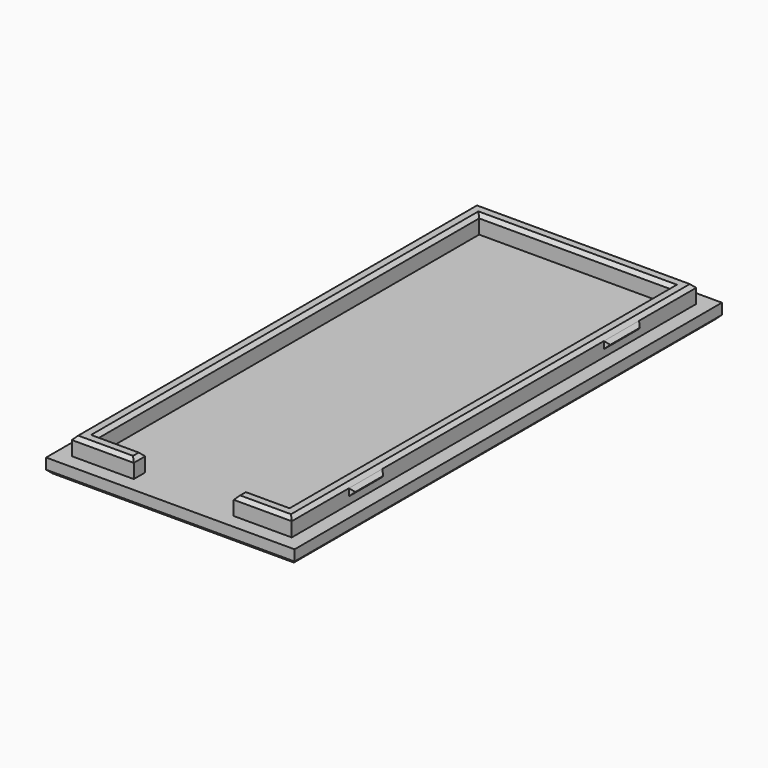
from build123d import *

# Parameters (mm, degrees)
F1_W     = 2
F1_H     = 6.165323171
F1_H_2   = 5.8635988384
F1_H_3   = 38.7710779905
F1_W_2   = 14
F1_H_4   = 2
F1_W_3   = 26.8
F1_H_5   = 8
F1_W_4   = 0.5
F2_DEPTH = 2
F3_START = 1
F3_DEPTH = 3.5
F4_START = 3
F4_DEPTH = 1
F5_SIZE  = 0.49999


# Not quite as in the source:
# - a fillet or chamfer is up to 0.001 mm smaller than in the source, because OpenCascade refuses the exact size


with BuildPart() as f2:
    # F1 (on Top) → F2 (new body)
    with BuildSketch(Plane.XY):
        Polygon((16.0419130247, 37.7546238333), (-14.7580869753, 37.7546238333), (-14.7580869753, 27.7546238333), (-12.7580869753, 27.7546238333), (-12.7580869753, 35.7546238333), (14.0419130247, 35.7546238333), (14.0419130247, 27.7546238333), (16.0419130247, 27.7546238333), align=None)
        Polygon((-12.7580869753, -23.0453761667), (-14.7580869753, -23.0453761667), (-14.7580869753, -26.0453761667), (-14.7580869753, -33.0453761667), (-6.0801735182, -33.0453761667), (-6.0801735182, -31.0453761667), (-12.7580869753, -31.0453761667), align=None)
        with Locations((-13.7580869753, 24.6719622478)):
            Rectangle(F1_W, F1_H)
        with Locations((-13.7580869753, -20.1135767475)):
            Rectangle(F1_W, F1_H_2)
        Polygon((-12.7580869753, 21.5893006623), (-14.7580869753, 21.5893006623), (-14.7580869753, -3.2453761667), (-14.7580869753, -17.1817773283), (-12.7580869753, -17.1817773283), align=None)
        with Locations((15.0419130247, 2.203761667)):
            Rectangle(F1_W, F1_H_3)
        with Locations((15.0419130247, -20.1135767475)):
            Rectangle(F1_W, F1_H_2)
        Polygon((16.0419130247, -33.0453761667), (16.0419130247, -23.0453761667), (14.0419130247, -23.0453761667), (14.0419130247, -31.0453761667), (7.9198264818, -31.0453761667), (7.9198264818, -33.0453761667), align=None)
        with Locations((15.0419130247, 24.6719622478)):
            Rectangle(F1_W, F1_H)
        Polygon((-14.7580869753, -26.0453761667), (-16.7580869753, -26.0453761667), (-16.7580869753, -35.0453761667), (-6.0801735182, -35.0453761667), (-6.0801735182, -33.0453761667), (-14.7580869753, -33.0453761667), align=None)
        with Locations((0.9198264818, -32.0453761667)):
            Rectangle(F1_W_2, F1_H_4)
        with Locations((0.9198264818, -34.0453761667)):
            Rectangle(F1_W_2, F1_H_4)
        with Locations((0.6419130247, 24.6719622478)):
            Rectangle(F1_W_3, F1_H)
        with Locations((0.6419130247, 2.203761667)):
            Rectangle(F1_W_3, F1_H_3)
        Polygon((14.0419130247, -23.0453761667), (-12.7580869753, -23.0453761667), (-12.7580869753, -31.0453761667), (-6.0801735182, -31.0453761667), (7.9198264818, -31.0453761667), (14.0419130247, -31.0453761667), align=None)
        Polygon((-14.7580869753, 27.7546238333), (-14.7580869753, 37.7546238333), (16.0419130247, 37.7546238333), (16.0419130247, 27.7546238333), (16.5419130247, 27.7546238333), (16.5419130247, 21.5893006623), (16.0419130247, 21.5893006623), (16.0419130247, -17.1817773283), (16.5419130247, -17.1817773283), (16.5419130247, -23.0453761667), (16.0419130247, -23.0453761667), (16.0419130247, -33.0453761667), (7.9198264818, -33.0453761667), (7.9198264818, -35.0453761667), (18.0419130247, -35.0453761667), (18.0419130247, 39.7546238333), (-16.7580869753, 39.7546238333), (-16.7580869753, -3.2453761667), (-14.7580869753, -3.2453761667), (-14.7580869753, 21.5893006623), (-15.2580869753, 21.5893006623), (-15.2580869753, 27.7546238333), align=None)
        with Locations((0.6419130247, 31.7546238333)):
            Rectangle(F1_W_3, F1_H_5)
        Polygon((-14.7580869753, -17.1817773283), (-14.7580869753, -3.2453761667), (-16.7580869753, -3.2453761667), (-16.7580869753, -26.0453761667), (-14.7580869753, -26.0453761667), (-14.7580869753, -23.0453761667), (-15.2580869753, -23.0453761667), (-15.2580869753, -17.1817773283), align=None)
        with Locations((0.6419130247, -20.1135767475)):
            Rectangle(F1_W_3, F1_H_2)
        with Locations((-15.0080869753, -20.1135767475)):
            Rectangle(F1_W_4, F1_H_2)
        with Locations((-15.0080869753, 24.6719622478)):
            Rectangle(F1_W_4, F1_H)
        with Locations((16.2919130247, -20.1135767475)):
            Rectangle(F1_W_4, F1_H_2)
        with Locations((16.2919130247, 24.6719622478)):
            Rectangle(F1_W_4, F1_H)
    extrude(amount=F2_DEPTH)

    # F1 (on Top) → F3 (join)
    with BuildSketch(Plane.XY.offset(F3_START)):
        Polygon((16.0419130247, 37.7546238333), (-14.7580869753, 37.7546238333), (-14.7580869753, 27.7546238333), (-12.7580869753, 27.7546238333), (-12.7580869753, 35.7546238333), (14.0419130247, 35.7546238333), (14.0419130247, 27.7546238333), (16.0419130247, 27.7546238333), align=None)
        with Locations((-13.7580869753, 24.6719622478)):
            Rectangle(F1_W, F1_H)
        with Locations((15.0419130247, 24.6719622478)):
            Rectangle(F1_W, F1_H)
        with Locations((15.0419130247, 2.203761667)):
            Rectangle(F1_W, F1_H_3)
        Polygon((-12.7580869753, 21.5893006623), (-14.7580869753, 21.5893006623), (-14.7580869753, -3.2453761667), (-14.7580869753, -17.1817773283), (-12.7580869753, -17.1817773283), align=None)
        with Locations((15.0419130247, -20.1135767475)):
            Rectangle(F1_W, F1_H_2)
        Polygon((16.0419130247, -33.0453761667), (16.0419130247, -23.0453761667), (14.0419130247, -23.0453761667), (14.0419130247, -31.0453761667), (7.9198264818, -31.0453761667), (7.9198264818, -33.0453761667), align=None)
        Polygon((-12.7580869753, -23.0453761667), (-14.7580869753, -23.0453761667), (-14.7580869753, -26.0453761667), (-14.7580869753, -33.0453761667), (-6.0801735182, -33.0453761667), (-6.0801735182, -31.0453761667), (-12.7580869753, -31.0453761667), align=None)
        with Locations((-13.7580869753, -20.1135767475)):
            Rectangle(F1_W, F1_H_2)
    extrude(amount=F3_DEPTH)

    # F1 (on Top) → F4 (join)
    with BuildSketch(Plane.XY.offset(F4_START)):
        with Locations((-15.0080869753, 24.6719622478)):
            Rectangle(F1_W_4, F1_H)
        with Locations((-15.0080869753, -20.1135767475)):
            Rectangle(F1_W_4, F1_H_2)
        with Locations((16.2919130247, -20.1135767475)):
            Rectangle(F1_W_4, F1_H_2)
        with Locations((16.2919130247, 24.6719622478)):
            Rectangle(F1_W_4, F1_H)
    extrude(amount=F4_DEPTH)

    # F5 (size 0.5 in the source; OpenCascade refuses exactly that, so slightly less here)
    f5_edges = [f2.edges().sort_by_distance(p)[0] for p in [
        (0.641913, -35.045376, 0),
        (18.041913, 2.354624, 0),
        (0.641913, 39.754624, 0),
        (-16.758087, 2.354624, 0),
        (16.541913, -23.045376, 3.5),
        (16.541913, -17.181777, 3.5),
        (16.541913, -20.113577, 3),
        (16.541913, -20.113577, 4),
        (16.541913, 21.589301, 3.5),
        (16.541913, 27.754624, 3.5),
        (16.541913, 24.671962, 3),
        (16.541913, 24.671962, 4),
        (-15.258087, 27.754624, 3.5),
        (-15.258087, 21.589301, 3.5),
        (-15.258087, 24.671962, 3),
        (-15.258087, 24.671962, 4),
        (-15.258087, -17.181777, 3.5),
        (-15.258087, -23.045376, 3.5),
        (-15.258087, -20.113577, 3),
        (-15.258087, -20.113577, 4),
        (0.641913, 37.754624, 4.5),
        (-14.758087, 2.354624, 4.5),
        (-10.41913, -33.045376, 4.5),
        (-6.080174, -32.045376, 4.5),
        (-9.41913, -31.045376, 4.5),
        (-12.758087, 2.354624, 4.5),
        (0.641913, 35.754624, 4.5),
        (14.041913, 2.354624, 4.5),
        (10.98087, -31.045376, 4.5),
        (7.919826, -32.045376, 4.5),
        (11.98087, -33.045376, 4.5),
        (16.041913, 2.354624, 4.5),
    ]]
    chamfer(f5_edges, length=F5_SIZE)


solid = f2.part
